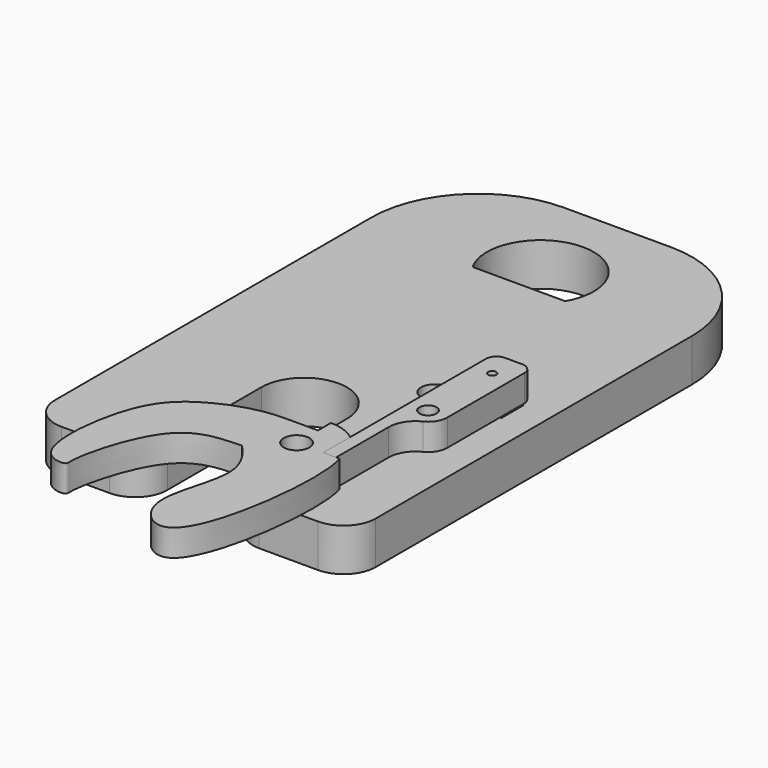
from build123d import *

# Parameters (mm, degrees)
F0_R     = 1.524
F1_DEPTH = 3.175
F2_R     = 0.635
F3_DEPTH = 5.08
F4_R     = 1.016
F4_R_2   = 0.4765946888
F5_DEPTH = 3.175
F6_D     = 1.016
F8_DEPTH = 25.4


with BuildPart() as f1:
    # F0 (on Top) → F1 (new body)
    with BuildSketch(Plane.XY):
        with BuildLine():
            add(Edge.make_bspline(
                [(4.0146798487, 4.0146798487), (4.1965253446, 3.8388911287), (8.6034145204, -0.4632855785), (2.7081005667, -9.8256704348), (11.7725199973, -17.5553609081), (14.1365779009, 3.6148799922), (12.7186926547, 7.62)],
                knots=[0.342546698, 0.342546698, 0.342546698, 0.342546698, 0.4592804701, 0.6325061967, 0.7529179928, 1, 1, 1, 1], degree=3))
            Line((12.7186926547, 7.62), (10.795, 7.62))
            Line((10.795, 7.62), (10.795, 11.6094914196))
            ThreePointArc((10.795, 11.6094914196), (9.3015879683, 12.4334113363), (7.62, 12.7186926547))
            Line((7.62, 12.7186926547), (7.62, 10.795))
            Line((7.62, 10.795), (3.6305085804, 10.795))
            add(Edge.make_bspline(
                [(-9.8462747246, -2.5595309993), (-9.7056248656, -0.6525965961), (-8.5851336869, 4.887523046), (-4.9223199156, 8.8010582074), (0.6214204647, 10.795), (3.6305085804, 10.795)],
                knots=[0.5944478908, 0.5944478908, 0.5944478908, 0.5944478908, 0.6806042793, 0.8326685389, 1, 1, 1, 1], degree=3))
            add(Edge.make_bspline(
                [(-9.8462747246, -2.5595309993), (-8.3692950914, 1.0159390836), (-1.2709087492, 7.2679963496), (3.9839462531, 4.0422517138), (3.9949946041, 4.0337094316), (4.0146798487, 4.0146798487)],
                knots=[0.0522687231, 0.0522687231, 0.0522687231, 0.0522687231, 0.2064144516, 0.3299099657, 0.342546698, 0.342546698, 0.342546698, 0.342546698], degree=3))
        make_face()
        with Locations((7.62, 7.62)):
            Circle(F0_R, mode=Mode.SUBTRACT)
        with BuildLine():
            add(Edge.make_bspline(
                [(4.0146798487, 4.0146798487), (1.5786877312, 3.9404286991), (-3.8406877482, 3.7898553775), (-6.77720019, -7.7849709454), (-6.196463978, -9.2958597248), (-9.5973471823, -8.9863377062), (-10.0193170502, -4.9056432962), (-9.8462747246, -2.5595309993)],
                knots=[0, 0, 0, 0, 0.1532538956, 0.3403377332, 0.3978065221, 0.4884491935, 0.5944478908, 0.5944478908, 0.5944478908, 0.5944478908], degree=3))
            add(Edge.make_bspline(
                [(-9.8462747246, -2.5595309993), (-8.3692950914, 1.0159390836), (-1.2709087492, 7.2679963496), (3.9839462531, 4.0422517138), (3.9949946041, 4.0337094316), (4.0146798487, 4.0146798487)],
                knots=[0.0522687231, 0.0522687231, 0.0522687231, 0.0522687231, 0.2064144516, 0.3299099657, 0.342546698, 0.342546698, 0.342546698, 0.342546698], degree=3))
        make_face()
    extrude(amount=F1_DEPTH)


with BuildPart() as f3:
    # F2 (on Top) → F3 (new body)
    with BuildSketch(Plane.XY):
        with BuildLine():
            Line((6.35, 64.77), (-6.35, 64.77))
            ThreePointArc((-6.35, 64.77), (-15.3302561211, 61.0502561211), (-19.05, 52.07))
            Line((-19.05, 52.07), (-19.05, 5.08))
            ThreePointArc((-19.05, 5.08), (-17.9340768363, 2.3859231637), (-15.24, 1.27))
            Line((-15.24, 1.27), (-9.525, 1.27))
            ThreePointArc((-9.525, 1.27), (-6.8309231637, 2.3859231637), (-5.715, 5.08))
            Line((-5.715, 5.08), (-5.715, 19.05))
            ThreePointArc((-5.715, 19.05), (-0.635, 24.13), (4.445, 19.05))
            Line((4.445, 19.05), (4.445, 5.08))
            ThreePointArc((4.445, 5.08), (5.5609231637, 2.3859231637), (8.255, 1.27))
            Line((8.255, 1.27), (15.24, 1.27))
            ThreePointArc((15.24, 1.27), (17.9340768363, 2.3859231637), (19.05, 5.08))
            Line((19.05, 5.08), (19.05, 52.07))
            ThreePointArc((19.05, 52.07), (15.3302561211, 61.0502561211), (6.35, 64.77))
        make_face()
        with Locations((7.62, 7.62)):
            Circle(F2_R, mode=Mode.SUBTRACT)
        with BuildLine():
            ThreePointArc((-5.499261314, 50.165), (0, 59.69), (5.499261314, 50.165))
            Line((5.499261314, 50.165), (-5.499261314, 50.165))
        make_face(mode=Mode.SUBTRACT)
    extrude(amount=-F3_DEPTH)

    # F6 (through all)
    with Locations(Plane.XY):
        with Locations((13.081, 20.32)):
            Hole(F6_D / 2)

    # F7 (on face) → F8 (cut)
    with BuildSketch(Plane.XY):
        with BuildLine():
            Line((15.5435356842, 28.1201432546), (15.5435356842, 31.4043808392))
            ThreePointArc((15.5435356842, 31.4043808392), (10.8526970709, 31.4538334208), (6.542203401, 29.6028723799))
            ThreePointArc((6.542203401, 29.6028723799), (6.1585518853, 27.3908316899), (8.3705925754, 27.0071801742))
            ThreePointArc((8.3705925754, 27.0071801742), (11.826845486, 28.4029087118), (15.5435356842, 28.1201432546))
        make_face()
    extrude(amount=-F8_DEPTH, mode=Mode.SUBTRACT)


with BuildPart() as f5:
    # F4 (on face) → F5 (new body)
    with BuildSketch(Plane.XY):
        with BuildLine():
            Line((10.795, 31.75), (10.795, 7.62))
            Line((10.795, 7.62), (12.319, 7.62))
            Line((12.319, 7.62), (12.319, 15.4210254134))
            ThreePointArc((12.319, 15.4210254134), (12.7981833657, 17.09828439), (14.0910930233, 18.2692664521))
            ThreePointArc((14.0910930233, 18.2692664521), (15.0219879767, 19.1123735369), (15.367, 20.32))
            Line((15.367, 20.32), (15.367, 31.75))
            ThreePointArc((15.367, 31.75), (14.9950256121, 32.6480256121), (14.097, 33.02))
            Line((14.097, 33.02), (12.065, 33.02))
            ThreePointArc((12.065, 33.02), (11.1669743879, 32.6480256121), (10.795, 31.75))
        make_face()
        with Locations((13.081, 20.32)):
            Circle(F4_R, mode=Mode.SUBTRACT)
        with Locations((13.081, 29.845)):
            Circle(F4_R_2, mode=Mode.SUBTRACT)
    extrude(amount=F5_DEPTH)


solid = Compound([f1.part, f3.part, f5.part])
